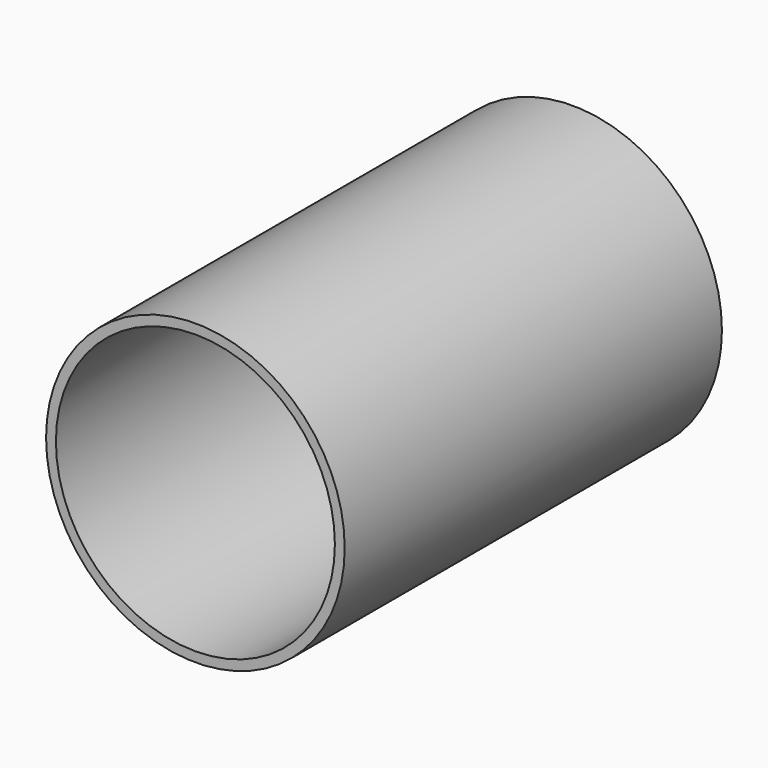
from build123d import *

# Parameters (mm, degrees)
F0_R     = 38
F0_R_2   = 35.5
F1_DEPTH = 120


# Not quite as in the source:
# - the program builds the solid bodies; features that only make, move or delete a surface that nothing else refers to are left out


with BuildPart() as f1:
    # F0 (on Front) → F1 (new body)
    with BuildSketch(Plane.XZ):
        Circle(F0_R)
        Circle(F0_R_2, mode=Mode.SUBTRACT)
    extrude(amount=F1_DEPTH)


solid = f1.part
